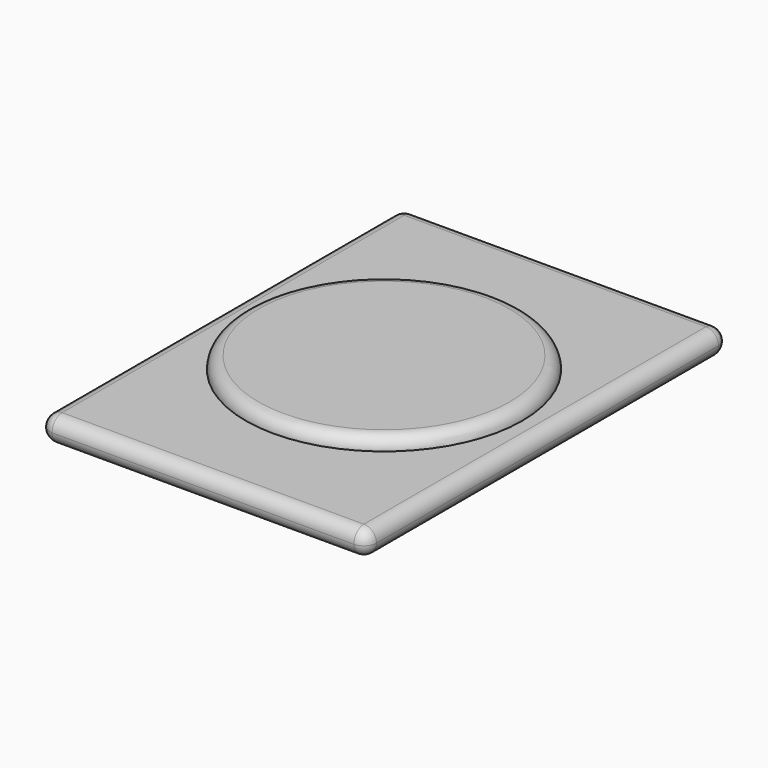
from build123d import *

# Parameters (mm, degrees)
F0_W     = 13
F0_H     = 18
F1_DEPTH = 1
F2_R     = 5.5
F3_DEPTH = 0.5
F4_R     = 0.49999


# Not quite as in the source:
# - a fillet or chamfer is up to 0.001 mm smaller than in the source, because OpenCascade refuses the exact size


with BuildPart() as f1:
    # F0 (on Top) → F1 (new body)
    with BuildSketch(Plane.XY):
        with Locations((-28.8841596369, 33.0711239949)):
            Rectangle(F0_W, F0_H)
    extrude(amount=F1_DEPTH)

    # F2 (on face) → F3 (join)
    with BuildSketch(Plane.XY.offset(1)):
        with Locations((-28.8841596369, 33.0711239949)):
            Circle(F2_R)
    extrude(amount=F3_DEPTH)

    # F4 (radius 0.5 in the source; OpenCascade refuses exactly that, so slightly less here)
    f4_edges = [f1.edges().sort_by_distance(p)[0] for p in [
        (-28.88416, 42.071124, 1),
        (-28.88416, 42.071124, 0),
        (-35.38416, 33.071124, 1),
        (-22.38416, 33.071124, 1),
        (-28.88416, 24.071124, 1),
        (-34.38416, 33.071124, 1.5),
        (-22.38416, 42.071124, 0.5),
        (-22.38416, 33.071124, 0),
        (-35.38416, 33.071124, 0),
        (-28.88416, 24.071124, 0),
        (-22.38416, 24.071124, 0.5),
        (-35.38416, 24.071124, 0.5),
        (-35.38416, 42.071124, 0.5),
    ]]
    fillet(f4_edges, radius=F4_R)


solid = f1.part
